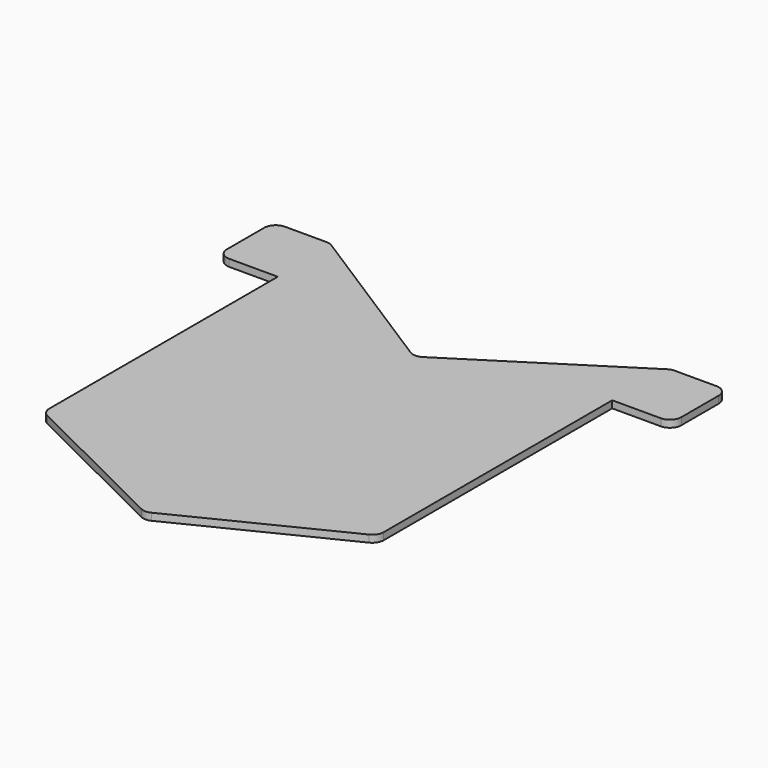
from build123d import *

# Parameters (mm, degrees)
F1_DEPTH = 3.175
F2_R     = 5.08
F3_R     = 5.08


# Not quite as in the source:
# - two fillets or chamfers of one size are made in one step


with BuildPart() as f1:
    # F0 (on Top) → F1 (new body)
    with BuildSketch(Plane.XY):
        Polygon((0, -34.215349704), (-53.7331599414, 0), (-75.9016672165, 14.1161106039), (-101.0106563997, 14.1161106039), (-101.0106563997, 7.5655808932), (-101.0106563997, 0), (-101.0106563997, -16.8134532869), (-74.3406563997, -16.8134532869), (-74.3406563997, -43.2344191068), (-74.3406563997, -119.4344191068), (-74.3406563997, -146.9356715679), (0, -183.8173121214), align=None)
        Polygon((53.7331599414, 0), (0, -34.215349704), (0, -183.8173121214), (74.3406563997, -146.9356715679), (74.3406563997, -119.4344191068), (74.3406563997, -43.2344191068), (74.3406563997, -16.8134532869), (101.0106563997, -16.8134532869), (101.0106563997, 14.1161106039), (75.9016672165, 14.1161106039), align=None)
    extrude(amount=F1_DEPTH)

    # F2
    f2_edges = [f1.edges().sort_by_distance(p)[0] for p in [
        (0, -34.21535, 1.5875),
    ]]
    fillet(f2_edges, radius=F2_R)

    # F3
    f3_edges = [f1.edges().sort_by_distance(p)[0] for p in [
        (-74.340656, -146.935672, 1.5875),
        (0, -183.817312, 1.5875),
        (74.340656, -146.935672, 1.5875),
        (-75.901667, 14.116111, 1.5875),
        (-101.010656, 14.116111, 1.5875),
        (75.901667, 14.116111, 1.5875),
        (-101.010656, -16.813453, 1.5875),
        (101.010656, 14.116111, 1.5875),
        (101.010656, -16.813453, 1.5875),
    ]]
    fillet(f3_edges, radius=F3_R)


solid = f1.part
